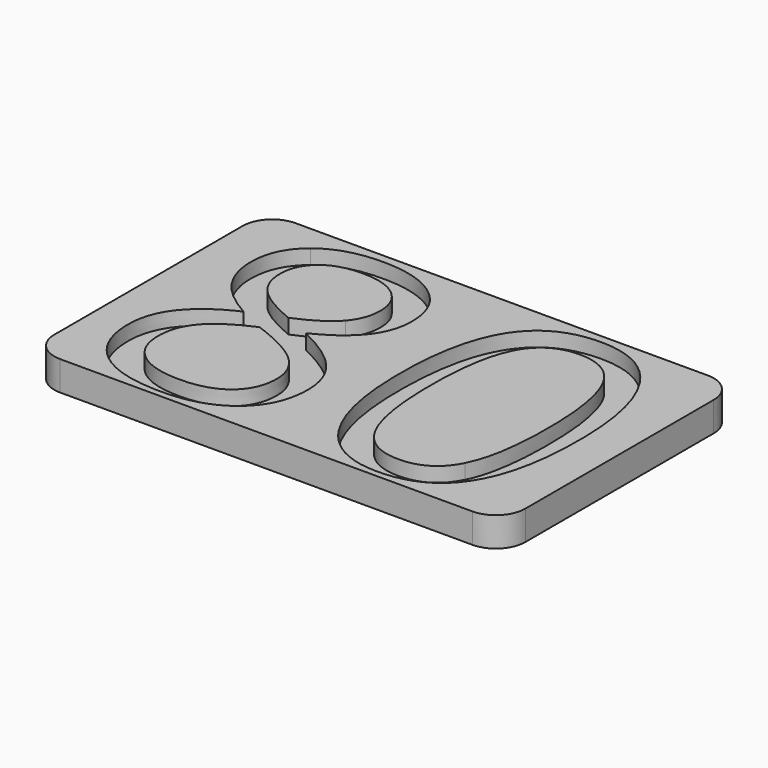
from build123d import *

# Parameters (mm, degrees)
F1_DEPTH     = 6.35
F0_TEXT_SIZE = 82.2117329737
F2_DEPTH     = 3.175


# Not quite as in the source:
# - Text() gives the source's letters only with a copy of the font that has no kerning and outlines rounded to 1/6400 em; it was checked with that copy


with BuildPart() as f1:
    # F0 (on Top) → F1 (new body)
    with BuildSketch(Plane.XY):
        with BuildLine():
            Line((44.45, 31.75), (-44.45, 31.75))
            ThreePointArc((-44.45, 31.75), (-48.9401280605, 29.8901280605), (-50.8, 25.4))
            Line((-50.8, 25.4), (-50.8, -25.4))
            ThreePointArc((-50.8, -25.4), (-48.9401280605, -29.8901280605), (-44.45, -31.75))
            Line((-44.45, -31.75), (44.45, -31.75))
            ThreePointArc((44.45, -31.75), (48.9401280605, -29.8901280605), (50.8, -25.4))
            Line((50.8, -25.4), (50.8, 25.4))
            ThreePointArc((50.8, 25.4), (48.9401280605, 29.8901280605), (44.45, 31.75))
        make_face()
        with BuildLine():
            add(Edge.make_bspline(
                [(-36.8090188806, 26.1355380984), (-32.0946898179, 29.9249851652), (-24.1818105192, 29.9249851652)],
                knots=[0, 0, 0, 1, 1, 1], degree=2))
            add(Edge.make_bspline(
                [(-24.1818105192, 29.9249851652), (-16.153320971, 29.9249851652), (-11.4582602832, 26.1933432232)],
                knots=[0, 0, 0, 1, 1, 1], degree=2))
            add(Edge.make_bspline(
                [(-11.4582602832, 26.1933432232), (-6.7631995954, 22.4617012812), (-6.7631995954, 15.8847626433)],
                knots=[0, 0, 0, 1, 1, 1], degree=2))
            add(Edge.make_bspline(
                [(-6.7631995954, 15.8847626433), (-6.7631995954, 11.5429554956), (-9.4479265003, 7.9718833446)],
                knots=[0, 0, 0, 1, 1, 1], degree=2))
            add(Edge.make_bspline(
                [(-9.4479265003, 7.9718833446), (-12.1326534053, 4.4008111935), (-18.0416217127, 1.4720182063)],
                knots=[0, 0, 0, 1, 1, 1], degree=2))
            add(Edge.make_bspline(
                [(-18.0416217127, 1.4720182063), (-10.8994774107, -1.9449069454), (-7.8871881322, -5.6958172623)],
                knots=[0, 0, 0, 1, 1, 1], degree=2))
            add(Edge.make_bspline(
                [(-7.8871881322, -5.6958172623), (-4.8748988537, -9.4467275792), (-4.8748988537, -14.3922771409)],
                knots=[0, 0, 0, 1, 1, 1], degree=2))
            add(Edge.make_bspline(
                [(-4.8748988537, -14.3922771409), (-4.8748988537, -21.6885684423), (-9.9745954147, -26.0496439649)],
                knots=[0, 0, 0, 1, 1, 1], degree=2))
            add(Edge.make_bspline(
                [(-9.9745954147, -26.0496439649), (-15.0742919757, -30.4107194875), (-23.937744437, -30.4107194875)],
                knots=[0, 0, 0, 1, 1, 1], degree=2))
            add(Edge.make_bspline(
                [(-23.937744437, -30.4107194875), (-33.3278658125, -30.4107194875), (-38.3890256237, -26.2937100472)],
                knots=[0, 0, 0, 1, 1, 1], degree=2))
            add(Edge.make_bspline(
                [(-38.3890256237, -26.2937100472), (-43.4501854349, -22.1767006069), (-43.4501854349, -14.6234976399)],
                knots=[0, 0, 0, 1, 1, 1], degree=2))
            add(Edge.make_bspline(
                [(-43.4501854349, -14.6234976399), (-43.4501854349, -4.5525603506), (-31.169807822, 1.0738051247)],
                knots=[0, 0, 0, 1, 1, 1], degree=2))
            add(Edge.make_bspline(
                [(-31.169807822, 1.0738051247), (-36.7062542144, 4.1952818611), (-39.1148010789, 7.8305819285)],
                knots=[0, 0, 0, 1, 1, 1], degree=2))
            add(Edge.make_bspline(
                [(-39.1148010789, 7.8305819285), (-41.5233479434, 11.465881996), (-41.5233479434, 15.961836143)],
                knots=[0, 0, 0, 1, 1, 1], degree=2))
            add(Edge.make_bspline(
                [(-41.5233479434, 15.961836143), (-41.5233479434, 22.3460910317), (-36.8090188806, 26.1355380984)],
                knots=[0, 0, 0, 1, 1, 1], degree=2))
        make_face(mode=Mode.SUBTRACT)
        with BuildLine():
            add(Edge.make_bspline(
                [(37.335687795, 22.2625947404), (42.29408294, 14.5102852326), (42.29408294, -0.1722164531)],
                knots=[0, 0, 0, 1, 1, 1], degree=2))
            add(Edge.make_bspline(
                [(42.29408294, -0.1722164531), (42.29408294, -15.3942326365), (37.496257586, -22.902476062)],
                knots=[0, 0, 0, 1, 1, 1], degree=2))
            add(Edge.make_bspline(
                [(37.496257586, -22.902476062), (32.698432232, -30.4107194875), (22.8201786918, -30.4107194875)],
                knots=[0, 0, 0, 1, 1, 1], degree=2))
            add(Edge.make_bspline(
                [(22.8201786918, -30.4107194875), (13.3529838166, -30.4107194875), (8.4138570465, -22.7226378962)],
                knots=[0, 0, 0, 1, 1, 1], degree=2))
            add(Edge.make_bspline(
                [(8.4138570465, -22.7226378962), (3.4747302765, -15.0345563048), (3.4747302765, -0.1722164531)],
                knots=[0, 0, 0, 1, 1, 1], degree=2))
            add(Edge.make_bspline(
                [(3.4747302765, -0.1722164531), (3.4747302765, 15.1525643965), (8.2532872556, 22.5837343223)],
                knots=[0, 0, 0, 1, 1, 1], degree=2))
            add(Edge.make_bspline(
                [(8.2532872556, 22.5837343223), (13.0318442347, 30.0149042481), (22.8201786918, 30.0149042481)],
                knots=[0, 0, 0, 1, 1, 1], degree=2))
            add(Edge.make_bspline(
                [(22.8201786918, 30.0149042481), (32.37729265, 30.0149042481), (37.335687795, 22.2625947404)],
                knots=[0, 0, 0, 1, 1, 1], degree=2))
        make_face(mode=Mode.SUBTRACT)
    extrude(amount=F1_DEPTH)



with BuildPart() as f1b:
    # F0 (on Top) → F1, piece 2 (new body)
    with BuildSketch(Plane.XY):
        with BuildLine():
            add(Edge.make_bspline(
                [(-16.2496628456, 22.127716116), (-19.1591874579, 24.5169946055), (-24.2588840189, 24.5169946055)],
                knots=[0, 0, 0, 1, 1, 1], degree=2))
            add(Edge.make_bspline(
                [(-24.2588840189, 24.5169946055), (-29.2815070802, 24.5169946055), (-32.1332265678, 22.1084477411)],
                knots=[0, 0, 0, 1, 1, 1], degree=2))
            add(Edge.make_bspline(
                [(-32.1332265678, 22.1084477411), (-34.9849460553, 19.6999008766), (-34.9849460553, 15.6792333109)],
                knots=[0, 0, 0, 1, 1, 1], degree=2))
            add(Edge.make_bspline(
                [(-34.9849460553, 15.6792333109), (-34.9849460553, 11.9925509103), (-32.6149359407, 9.3399379636)],
                knots=[0, 0, 0, 1, 1, 1], degree=2))
            add(Edge.make_bspline(
                [(-32.6149359407, 9.3399379636), (-30.244925826, 6.6873250169), (-23.8606709373, 4.0411348618)],
                knots=[0, 0, 0, 1, 1, 1], degree=2))
            add(Edge.make_bspline(
                [(-23.8606709373, 4.0411348618), (-18.1186952124, 6.4432589346), (-15.7294167229, 9.2179049225)],
                knots=[0, 0, 0, 1, 1, 1], degree=2))
            add(Edge.make_bspline(
                [(-15.7294167229, 9.2179049225), (-13.3401382333, 11.9925509103), (-13.3401382333, 15.6792333109)],
                knots=[0, 0, 0, 1, 1, 1], degree=2))
            add(Edge.make_bspline(
                [(-13.3401382333, 15.6792333109), (-13.3401382333, 19.7384376264), (-16.2496628456, 22.127716116)],
                knots=[0, 0, 0, 1, 1, 1], degree=2))
        make_face()
    extrude(amount=F1_DEPTH)


with BuildPart() as f1c:
    # F0 (on Top) → F1, piece 3 (new body)
    with BuildSketch(Plane.XY):
        with BuildLine():
            add(Edge.make_bspline(
                [(-34.1756743088, -7.3400519218), (-36.8604012138, -10.4486830748), (-36.8604012138, -14.7904902225)],
                knots=[0, 0, 0, 1, 1, 1], degree=2))
            add(Edge.make_bspline(
                [(-36.8604012138, -14.7904902225), (-36.8604012138, -19.6075839514), (-33.5141267701, -22.298733648)],
                knots=[0, 0, 0, 1, 1, 1], degree=2))
            add(Edge.make_bspline(
                [(-33.5141267701, -22.298733648), (-30.1678523264, -24.9898833446), (-24.1047370196, -24.9898833446)],
                knots=[0, 0, 0, 1, 1, 1], degree=2))
            add(Edge.make_bspline(
                [(-24.1047370196, -24.9898833446), (-18.1186952124, -24.9898833446), (-14.785266352, -22.1767006069)],
                knots=[0, 0, 0, 1, 1, 1], degree=2))
            add(Edge.make_bspline(
                [(-14.785266352, -22.1767006069), (-11.4518374916, -19.3635178692), (-11.4518374916, -14.4693506406)],
                knots=[0, 0, 0, 1, 1, 1], degree=2))
            add(Edge.make_bspline(
                [(-11.4518374916, -14.4693506406), (-11.4518374916, -10.5771389076), (-14.5861598112, -7.5455812542)],
                knots=[0, 0, 0, 1, 1, 1], degree=2))
            add(Edge.make_bspline(
                [(-14.5861598112, -7.5455812542), (-17.7204821308, -4.5140236008), (-25.5049055968, -1.6623041133)],
                knots=[0, 0, 0, 1, 1, 1], degree=2))
            add(Edge.make_bspline(
                [(-25.5049055968, -1.6623041133), (-31.4909474039, -4.2314207687), (-34.1756743088, -7.3400519218)],
                knots=[0, 0, 0, 1, 1, 1], degree=2))
        make_face()
    extrude(amount=F1_DEPTH)


with BuildPart() as f1d:
    # F0 (on Top) → F1, piece 4 (new body)
    with BuildSketch(Plane.XY):
        with BuildLine():
            add(Edge.make_bspline(
                [(13.2309507755, 18.4346109238), (10.218661497, 12.6348300742), (10.218661497, -0.1722164531)],
                knots=[0, 0, 0, 1, 1, 1], degree=2))
            add(Edge.make_bspline(
                [(10.218661497, -0.1722164531), (10.218661497, -12.9792629804), (13.2309507755, -18.8240033715)],
                knots=[0, 0, 0, 1, 1, 1], degree=2))
            add(Edge.make_bspline(
                [(13.2309507755, -18.8240033715), (16.2432400539, -24.6687437626), (22.8201786918, -24.6687437626)],
                knots=[0, 0, 0, 1, 1, 1], degree=2))
            add(Edge.make_bspline(
                [(22.8201786918, -24.6687437626), (29.4870364127, -24.6687437626), (32.4736345246, -18.7469298719)],
                knots=[0, 0, 0, 1, 1, 1], degree=2))
            add(Edge.make_bspline(
                [(32.4736345246, -18.7469298719), (35.4602326365, -12.8251159811), (35.4602326365, -0.1722164531)],
                knots=[0, 0, 0, 1, 1, 1], degree=2))
            add(Edge.make_bspline(
                [(35.4602326365, -0.1722164531), (35.4602326365, 12.4678374916), (32.4736345246, 18.3511146325)],
                knots=[0, 0, 0, 1, 1, 1], degree=2))
            add(Edge.make_bspline(
                [(32.4736345246, 18.3511146325), (29.4870364127, 24.2343917734), (22.8201786918, 24.2343917734)],
                knots=[0, 0, 0, 1, 1, 1], degree=2))
            add(Edge.make_bspline(
                [(22.8201786918, 24.2343917734), (16.2432400539, 24.2343917734), (13.2309507755, 18.4346109238)],
                knots=[0, 0, 0, 1, 1, 1], degree=2))
        make_face()
    extrude(amount=F1_DEPTH)


with BuildPart() as f1_1:
    add(f1.part)

    add(f1b.part)  # F2 merges F1b

    add(f1c.part)  # F2 merges F1c

    add(f1d.part)  # F2 merges F1d
    # F0 (on Top) → F2 (join)
    with BuildSketch(Plane.XY):
        with Locations((-47.625, -29.6014477411)):
            Text('80', F0_TEXT_SIZE, font='Open Sans', text_align=(TextAlign.LEFT, TextAlign.BOTTOM))
    extrude(amount=F2_DEPTH)


solid = f1_1.part
